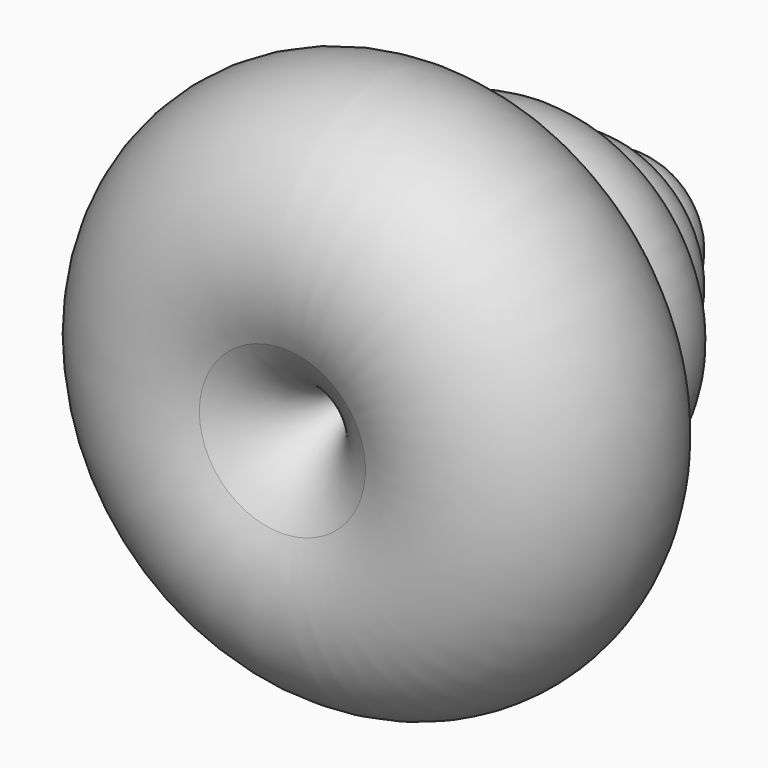
from build123d import *


with BuildPart() as f1:
    # F0 (on Top) → F1 (revolve)
    with BuildSketch(Plane.XY):
        with BuildLine():
            Line((-15.5635529785, 39.5905664053), (-15.7008221149, 45.8013020266))
            ThreePointArc((-15.7008221149, 45.8013020266), (-25.9890385476, 50.7794728031), (-32.1130069449, 41.1292607477))
            ThreePointArc((-32.1130069449, 41.1292607477), (-24.2210019432, 40.909417782), (-18.0212922533, 36.0210976578))
            ThreePointArc((-18.0212922533, 36.0210976578), (-16.5635800166, 37.6482636414), (-15.5635529785, 39.5905664053))
        make_face()
        with BuildLine():
            ThreePointArc((-18.0212922533, 36.0210976578), (-24.2210019432, 40.909417782), (-32.1130069449, 41.1292607477))
            ThreePointArc((-32.1130069449, 41.1292607477), (-26.564502454, 34.4444831281), (-18.0212922533, 36.0210976578))
        make_face()
        with BuildLine():
            ThreePointArc((-18.0212922533, 36.0210976578), (-26.564502454, 34.4444831281), (-32.1130069449, 41.1292607477))
            ThreePointArc((-32.1130069449, 41.1292607477), (-39.1241426865, 35.7916379536), (-40.8991822818, 27.16056178))
            ThreePointArc((-40.8991822818, 27.16056178), (-29.2726936854, 26.8876636908), (-19.9946800375, 19.875661609))
            ThreePointArc((-19.9946800375, 19.875661609), (-17.0029111772, 24.0677588183), (-15.9463685086, 29.1084013879))
            ThreePointArc((-15.9463685086, 29.1084013879), (-16.4762849853, 32.7170949973), (-18.0212922533, 36.0210976578))
        make_face()
        with BuildLine():
            ThreePointArc((-19.9946800375, 19.875661609), (-29.2726936854, 26.8876636908), (-40.8991822818, 27.16056178))
            ThreePointArc((-40.8991822818, 27.16056178), (-32.6294972412, 17.2550941542), (-19.9946800375, 19.875661609))
        make_face()
        with BuildLine():
            ThreePointArc((-19.9946800375, 19.875661609), (-32.6294972412, 17.2550941542), (-40.8991822818, 27.16056178))
            ThreePointArc((-40.8991822818, 27.16056178), (-52.6890937803, 16.9924939955), (-52.8846556294, 1.4247911728))
            ThreePointArc((-52.8846556294, 1.4247911728), (-37.541361976, 1.3866505854), (-24.2241672845, -6.2337457553))
            ThreePointArc((-24.2241672845, -6.2337457553), (-18.5824082634, 0.468287802), (-16.5576002259, 8.9916000143))
            ThreePointArc((-16.5576002259, 8.9916000143), (-17.4372866131, 14.6985325185), (-19.9946800375, 19.875661609))
        make_face()
        with BuildLine():
            ThreePointArc((-24.2241672845, -6.2337457553), (-37.541361976, 1.3866505854), (-52.8846556294, 1.4247911728))
            ThreePointArc((-52.8846556294, 1.4247911728), (-40.4017050576, -9.3175910109), (-24.2241672845, -6.2337457553))
        make_face()
        with BuildLine():
            ThreePointArc((-24.2241672845, -6.2337457553), (-40.4017050576, -9.3175910109), (-52.8846556294, 1.4247911728))
            ThreePointArc((-52.8846556294, 1.4247911728), (-73.332363025, -38.2282854938), (-31.7334887384, -54.3530764989))
            ThreePointArc((-31.7334887384, -54.3530764989), (-19.7286744278, -43.2972872449), (-15.2889961527, -27.5926605548))
            ThreePointArc((-15.2889961527, -27.5926605548), (-17.6128018618, -16.0163860616), (-24.2241672845, -6.2337457553))
        make_face()
    revolve(axis=Axis((-14.6278478205, -2.7453694493, 0), (0.0220965163, -0.9997558422, 0)))


solid = f1.part
